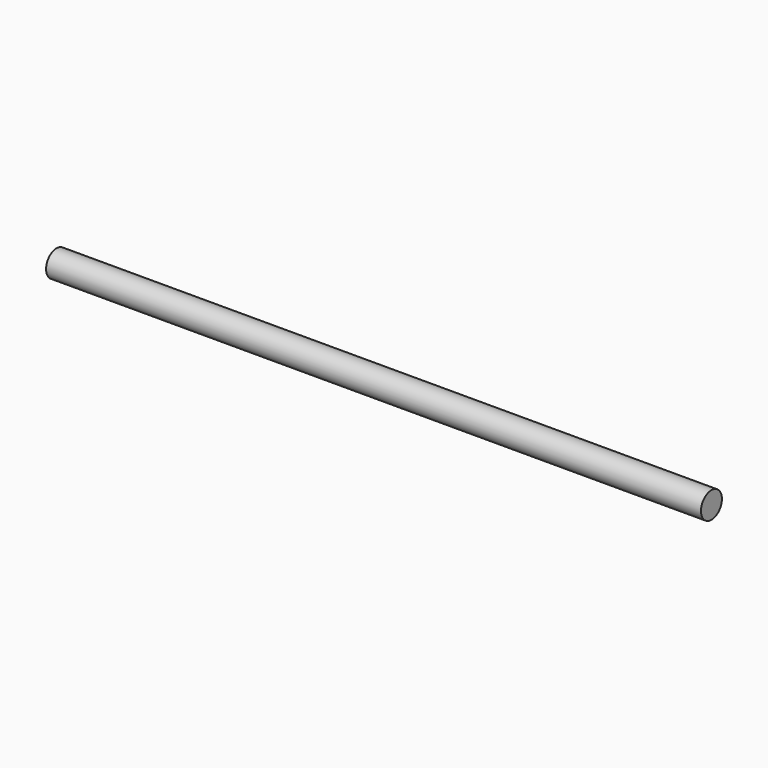
from build123d import *

# Parameters (mm, degrees)
F1_W = 150
F1_H = 3


# Not quite as in the source:
# - the program builds the solid bodies; features that only make, move or delete a surface that nothing else refers to are left out


with BuildPart() as f3:
    # F1 (on Front) → F3 (revolve)
    with BuildSketch(Plane.XZ):
        with Locations((184.567886591, 1.5)):
            Rectangle(F1_W, F1_H)
    revolve(axis=Axis((-24.9094008468, 0, 0), (-1, 0, 0)))


solid = f3.part
